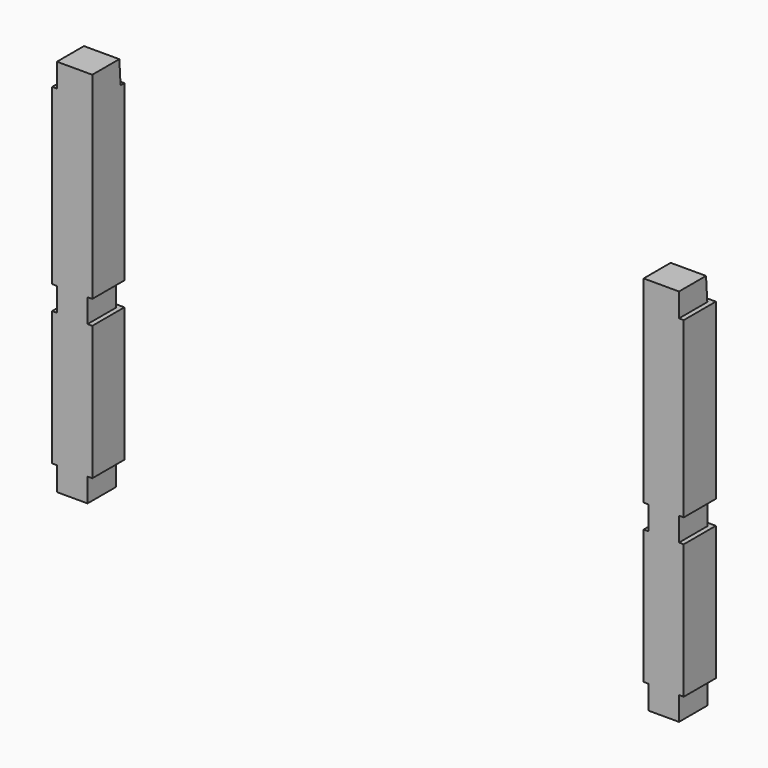
from build123d import *

# Parameters (mm, degrees)
F0_W      = 127
F0_H      = 127
F1_DEPTH  = 1200
F3_DEPTH  = 75
F5_START  = -500
F4_W      = 15
F4_H      = 127
F5_DEPTH  = 75
F7_DEPTH  = 127.001
F11_DEPTH = 75
F13_DEPTH = 75
F14_W     = 15
F14_H     = 75
F15_DEPTH = 127.001
F16_W     = 15
F16_H     = 75
F17_DEPTH = 127.001
F18_W     = 15
F18_H     = 75
F19_DEPTH = 1985.001
F20_W     = 15
F20_H     = 75
F21_DEPTH = 112.001
F22_R     = 11
F23_DEPTH = 25


# Not quite as in the source:
# - a feature names something its author has since deleted; it is built from what else it names


with BuildPart() as f1:
    # F0 (on Top) → F1 (new body)
    with BuildSketch(Plane.XY):
        with Locations((63.5, 63.5)):
            Rectangle(F0_W, F0_H)
    extrude(amount=F1_DEPTH)

    # F2 (on face) → F3 (cut)
    with BuildSketch(Plane.XY.offset(1200)):
        Polygon((0, 127), (0, 0), (15, 0), (15, 112), (127, 112), (127, 127), align=None)
    extrude(amount=-F3_DEPTH, mode=Mode.SUBTRACT)

    # F4 (on face) → F5 (cut)
    with BuildSketch(Plane(origin=(0, 0, 0), x_dir=(1, 0, 0), z_dir=(0, 0, -1)).offset(F5_START)):
        with Locations((7.5, -63.5)):
            Rectangle(F4_W, F4_H)
    extrude(amount=-F5_DEPTH, mode=Mode.SUBTRACT)

    # F6 (on face) → F7 (cut, through all)
    with BuildSketch(Plane.YZ.offset(127)):
        Polygon((112, 1125), (112, 1200), (107, 1200), align=None)
    extrude(amount=-F7_DEPTH, mode=Mode.SUBTRACT)


with BuildPart() as f9_1:
    # F9: instance of F1
    add(f1.part.mirror(Plane.YZ.offset(1000)))

    # F10 (on face) → F11 (cut)
    with BuildSketch(Plane(origin=(0, 0, 0), x_dir=(1, 0, 0), z_dir=(0, 0, -1))):
        Polygon((1873, -127), (2000, -127), (2000, 0), (1985, 0), (1985, -112), (1888, -112), (1888, 0), (1873, 0), align=None)
    extrude(amount=-F11_DEPTH, mode=Mode.SUBTRACT)

    # F16 (on face) → F17 (cut, through all)
    with BuildSketch(Plane.XZ):
        with Locations((1880.5, 537.5)):
            Rectangle(F16_W, F16_H)
    extrude(amount=-F17_DEPTH, mode=Mode.SUBTRACT)


with BuildPart() as f1_1:
    add(f1.part)

    # F12 (on face) → F13 (cut)
    with BuildSketch(Plane(origin=(0, 0, 0), x_dir=(1, 0, 0), z_dir=(0, 0, -1))):
        Polygon((0, -127), (127, -127), (127, 0), (112, 0), (112, -112), (15, -112), (15, 0), (0, 0), align=None)
    extrude(amount=-F13_DEPTH, mode=Mode.SUBTRACT)

    # F14 (on face) → F15 (cut, through all)
    with BuildSketch(Plane.XZ):
        with Locations((119.5, 537.5)):
            Rectangle(F14_W, F14_H)
    extrude(amount=-F15_DEPTH, mode=Mode.SUBTRACT)


with BuildPart() as f19_tool:
    # F18 (on face) → F19 (new body, through all)
    with BuildSketch(Plane(origin=(15, 0, 0), x_dir=(0, -1, 0), z_dir=(-1, 0, 0))):
        with Locations((-119.5, 537.5)):
            Rectangle(F18_W, F18_H)
    extrude(amount=-F19_DEPTH)


with BuildPart() as f1_2:
    add(f1_1.part)

    # F19: cut by f19_tool
    add(f19_tool.part, mode=Mode.SUBTRACT)

    # F20 (on face) → F21 (cut, through all)
    with BuildSketch(Plane(origin=(1888, 0, 0), x_dir=(0, -1, 0), z_dir=(-1, 0, 0))):
        with Locations((-119.5, 537.5)):
            Rectangle(F20_W, F20_H)
    extrude(amount=-F21_DEPTH, mode=Mode.SUBTRACT)


with BuildPart() as f9_1_1:
    add(f9_1.part)

    # F19: cut by f19_tool
    add(f19_tool.part, mode=Mode.SUBTRACT)

    # F22 (on face) → F23 (cut)
    with BuildSketch(Plane(origin=(0, 0, 0), x_dir=(1, 0, 0), z_dir=(0, 0, -1))):
        with Locations((1933, -67)):
            Circle(F22_R)
    extrude(amount=-F23_DEPTH, mode=Mode.SUBTRACT)


solid = Compound([f1_2.part, f9_1_1.part])
